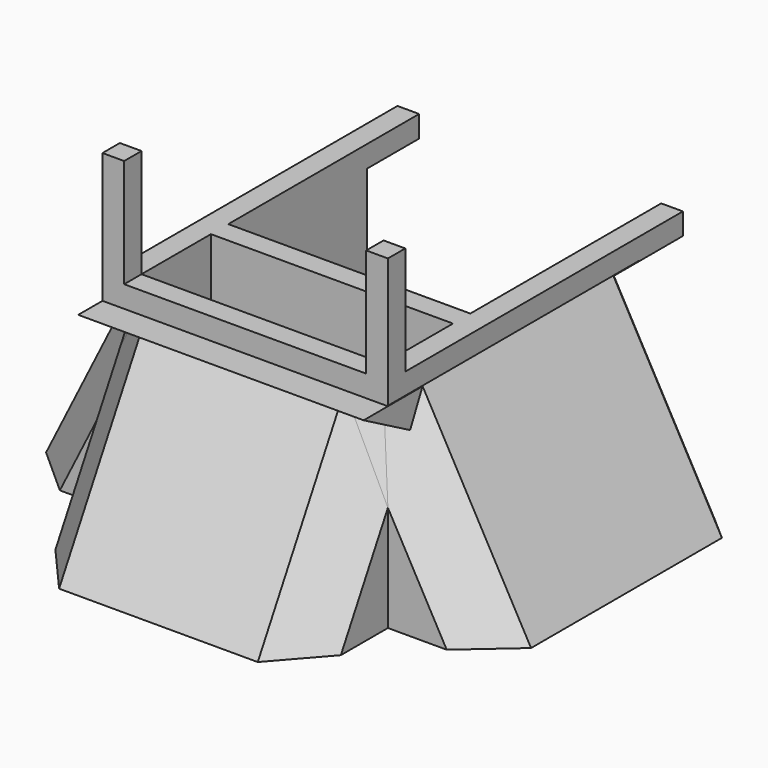
from build123d import *

# Parameters (mm, degrees)
F0_W          = 28.3464
F0_H          = 2.54
F0_W_2        = 2.54
F1_DEPTH      = 43.18
F2_W          = 28.3464
F2_H          = 10.16
F3_DEPTH      = 2.54
F2_W_2        = 2.54
F2_H_2        = 2.54
F4_DEPTH      = 12.7
F5_DEPTH      = 25.4
F6_W          = 33.4264
F6_H          = 22.86
F7_DEPTH      = 12.7
F9_W          = 35.56
F9_H          = 27.94
F10_DEPTH     = 25.4
F11_W         = 35.56
F11_H         = 22.86
F12_DEPTH     = 12.7
F14_W         = 36.8241928518
F14_H         = 28.1280204654
F15_DEPTH     = 25.4
F17_DEPTH     = 12.7
F19_W         = 36.3356121816
F19_H         = 38.6965835933
F20_DEPTH     = 25.4
F21_T4_DEPTH  = 37.4897748093
F21_T10_DEPTH = 37.4897748093
F22_T4_DEPTH  = 41.4622128931
F22_T9_DEPTH  = 41.4622128931
F22_T15_DEPTH = 39.215050137
F22_T21_DEPTH = 39.215050137
F22_T26_DEPTH = 13.1188216118
F23_T4_DEPTH  = 41.4622128931
F23_T9_DEPTH  = 41.4622128931
F23_T14_DEPTH = 39.215050137
F24_W         = 28.3464
F24_H         = 2.54
F25_DEPTH     = 25.4


# Not quite as in the source:
# - a fillet or chamfer that OpenCascade refuses, or shapes differently, is made with other operations: its cross-section is extruded or revolved along the edge and cut away or added


with BuildPart() as f1:
    # F0 (on Front) → F1 (new body)
    with BuildSketch(Plane.XZ):
        with Locations((16.7132, 1.27)):
            Rectangle(F0_W, F0_H)
        with Locations((1.27, 1.27)):
            Rectangle(F0_W_2, F0_H)
        with Locations((32.1564, 1.27)):
            Rectangle(F0_W_2, F0_H)
    extrude(amount=F1_DEPTH)

    # F2 (on face) → F3 (cut)
    with BuildSketch(Plane.XY.offset(2.54)):
        Polygon((30.8864, 0), (2.54, 0), (2.54, -7.62), (2.54, -27.94), (30.8864, -27.94), (30.8864, -7.62), align=None)
        with Locations((16.7132, -35.56)):
            Rectangle(F2_W, F2_H)
    extrude(amount=-F3_DEPTH, mode=Mode.SUBTRACT)

    # F2 (on face) → F4 (join)
    with BuildSketch(Plane.XY.offset(2.54)):
        with Locations((1.27, -41.91)):
            Rectangle(F2_W_2, F2_H_2)
        with Locations((32.1564, -41.91)):
            Rectangle(F2_W_2, F2_H_2)
    extrude(amount=F4_DEPTH)

    # F2 (on face) → F5 (join)
    with BuildSketch(Plane.XY.offset(2.54)):
        Polygon((2.54, -7.62), (0, -7.62), (0, -40.64), (2.54, -40.64), (2.54, -30.48), (2.54, -27.94), align=None)
        Polygon((33.4264, -7.62), (30.8864, -7.62), (30.8864, -27.94), (30.8864, -30.48), (30.8864, -40.64), (33.4264, -40.64), align=None)
        with Locations((16.7132, -41.91)):
            Rectangle(F2_W, F2_H_2)
        with Locations((1.27, -41.91)):
            Rectangle(F2_W_2, F2_H_2)
        with Locations((32.1564, -41.91)):
            Rectangle(F2_W_2, F2_H_2)
    extrude(amount=-F5_DEPTH)

    # F6 (on face) → F7 (join)
    with BuildSketch(Plane.XZ.offset(43.18)):
        with Locations((16.7132, -11.43)):
            Rectangle(F6_W, F6_H)
    extrude(amount=F7_DEPTH)

    # F9 (on 3pt) → F10 (cut)
    with BuildSketch(Plane(origin=(0, -32.9960377358, 18.3311320755), x_dir=(-1, 0, 0), z_dir=(0, 0.8741572761, -0.4856429312))):
        with Locations((-17.78, -36.665337096)):
            Rectangle(F9_W, F9_H)
    extrude(amount=-F10_DEPTH, mode=Mode.SUBTRACT)

    # F11 (on face) → F12 (join)
    with BuildSketch(Plane.YZ.offset(33.4264)):
        with Locations((-25.4, -11.43)):
            Rectangle(F11_W, F11_H)
    extrude(amount=F12_DEPTH)

    # F14 (on 3pt) → F15 (cut)
    with BuildSketch(Plane(origin=(25.5428150943, 0, 14.1904528302), x_dir=(0, -1, 0), z_dir=(-0.8741572761, 0, -0.4856429312))):
        with Locations((24.8448457569, -30.2426330745)):
            Rectangle(F14_W, F14_H)
    extrude(amount=-F15_DEPTH, mode=Mode.SUBTRACT)

    # F16 (on face) → F17 (join)
    with BuildSketch(Plane(origin=(0, 0, 0), x_dir=(0, -1, 0), z_dir=(-1, 0, 0))):
        Polygon((40.64, -22.86), (40.64, 2.54), (7.62, 2.54), (7.62, 0), (7.62, -22.86), align=None)
    extrude(amount=F17_DEPTH)

    # F19 (on 3pt) → F20 (cut)
    with BuildSketch(Plane(origin=(-1.016, 0, 0.508), x_dir=(0, -1, 0), z_dir=(-0.894427191, 0, 0.4472135955))):
        with Locations((25.5430552643, -17.0687864302)):
            Rectangle(F19_W, F19_H)
    extrude(amount=F20_DEPTH, mode=Mode.SUBTRACT)

    # F21: chamfer of 5.08 on 2 edges, made by hand


with BuildPart() as f21_tool2:
    # F21_s3 → F21_t4 (new body)
    with BuildSketch(Plane(origin=(0, -29.228474159, -52.6112534862), x_dir=(1, 0, 0), z_dir=(0, 0.4856429312, 0.8741572761))):
        with BuildLine():
            Line((-0.1436840979, -32.522427085), (5.2236840979, -37.8897952809))
            Line((5.2236840979, -37.8897952809), (5.2236840979, -37.9913952809))
            ThreePointArc((5.2236840979, -37.9913952809), (2.611842049, -37.8477111829), (0, -37.8477111829))
            Line((0, -37.8477111829), (-0.1016, -37.7461111829))
            ThreePointArc((-0.1016, -37.7461111829), (-0.1016, -35.134269134), (-0.2452840979, -32.522427085))
            Line((-0.2452840979, -32.522427085), (-0.1436840979, -32.522427085))
        make_face()
    extrude(amount=F21_T4_DEPTH)

    split(bisect_by=Plane.XY.offset(-22.86), keep=Keep.TOP)

    split(bisect_by=Plane.XZ.offset(40.64), keep=Keep.TOP)


with BuildPart() as f1_1:
    add(f1.part)

    # F21_t1: cut F21_tool2
    add(f21_tool2.part, mode=Mode.SUBTRACT)


with BuildPart() as f21_tool8:
    # F21_s9 → F21_t10 (new body)
    with BuildSketch(Plane(origin=(0, -11.0218300314, -19.8392940565), x_dir=(1, 0, 0), z_dir=(0, -0.4856429312, -0.8741572761))):
        with BuildLine():
            Line((33.5700840979, 32.522427085), (28.2027159021, 37.8897952809))
            Line((28.2027159021, 37.8897952809), (28.2027159021, 37.9913952809))
            ThreePointArc((28.2027159021, 37.9913952809), (30.814557951, 37.8477111829), (33.4264, 37.8477111829))
            Line((33.4264, 37.8477111829), (33.528, 37.7461111829))
            ThreePointArc((33.528, 37.7461111829), (33.528, 35.134269134), (33.6716840979, 32.522427085))
            Line((33.6716840979, 32.522427085), (33.5700840979, 32.522427085))
        make_face()
    extrude(amount=F21_T10_DEPTH)

    split(bisect_by=Plane.XZ.offset(43.18), keep=Keep.TOP)

    split(bisect_by=Plane.XY.offset(-22.86), keep=Keep.TOP)


with BuildPart() as f1_2:
    add(f1_1.part)

    # F21_t7: cut F21_tool8
    add(f21_tool8.part, mode=Mode.SUBTRACT)

    # F22: chamfer of 5.08 on 2 edges, made by hand


with BuildPart() as f22_tool2:
    # F22_s3 → F22_t4 (new body)
    with BuildSketch(Plane(origin=(-17.5264653053, 0, -35.0529306106), x_dir=(0, 1, 0), z_dir=(0.4472135955, 0, 0.894427191))):
        Polygon((-40.64, -3.9440774674), (-35.56, 1.1359225326), (-40.64, 1.1359225326), align=None)
    extrude(amount=F22_T4_DEPTH)

    split(bisect_by=Plane.YZ, keep=Keep.BOTTOM)


with BuildPart() as f1_3:
    add(f1_2.part)

    # F22_t1: cut F22_tool2
    add(f22_tool2.part, mode=Mode.SUBTRACT)


with BuildPart() as f22_tool7:
    # F22_s8 → F22_t9 (new body)
    with BuildSketch(Plane(origin=(-17.5264653053, 0, -35.0529306106), x_dir=(0, 1, 0), z_dir=(0.4472135955, 0, 0.894427191))):
        Polygon((-40.64, -3.9440774674), (-35.56, 1.1359225326), (-40.64, 1.1359225326), align=None)
    extrude(amount=F22_T9_DEPTH)

    split(bisect_by=Plane(origin=(-16.3330555915, -14.2776593863, 7.9320329924), x_dir=(0.6581451817, -0.7528910411, 0), z_dir=(-0.7071067812, -0.6181225378, 0.3434014099)), keep=Keep.TOP)

    split(bisect_by=Plane(origin=(0, -11.0218300314, -19.8392940565), x_dir=(1, 0, 0), z_dir=(0, -0.4856429312, -0.8741572761)), keep=Keep.TOP)


with BuildPart() as f1_4:
    add(f1_3.part)

    # F22_t6: cut F22_tool7
    add(f22_tool7.part, mode=Mode.SUBTRACT)


with BuildPart() as f22_tool13:
    # F22_s14 → F22_t15 (new body)
    with BuildSketch(Plane(origin=(26.9280968005, 0, -48.4705742409), x_dir=(0, 1, 0), z_dir=(-0.4856429312, 0, 0.8741572761))):
        Polygon((-38.1, -29.2199307745), (-43.18, -24.1399307745), (-43.18, -29.2199307745), align=None)
    extrude(amount=F22_T15_DEPTH)

    split(bisect_by=Plane(origin=(33.0462555918, -28.8876247736, 16.0486804298), x_dir=(0.6581451817, 0.7528910411, 0), z_dir=(0.7071067812, -0.6181225378, 0.3434014099)), keep=Keep.TOP)

    split(bisect_by=Plane(origin=(0, -11.0218300314, -19.8392940565), x_dir=(1, 0, 0), z_dir=(0, -0.4856429312, -0.8741572761)), keep=Keep.TOP)


with BuildPart() as f1_5:
    add(f1_4.part)

    # F22_t12: cut F22_tool13
    add(f22_tool13.part, mode=Mode.SUBTRACT)


with BuildPart() as f22_tool19:
    # F22_s20 → F22_t21 (new body)
    with BuildSketch(Plane(origin=(26.9280968005, 0, -48.4705742409), x_dir=(0, 1, 0), z_dir=(-0.4856429312, 0, 0.8741572761))):
        Polygon((-38.1, -29.2199307745), (-43.18, -24.1399307745), (-43.18, -29.2199307745), align=None)
    extrude(amount=F22_T21_DEPTH)

    split(bisect_by=Plane.YZ.offset(33.4264), keep=Keep.TOP)


with BuildPart() as f1_6:
    add(f1_5.part)

    # F22_t18: cut F22_tool19
    add(f22_tool19.part, mode=Mode.SUBTRACT)


with BuildPart() as f22_tool24:
    # F22_s25 → F22_t26 (new body)
    with BuildSketch(Plane(origin=(1.5125219245, 0, -2.7225394641), x_dir=(0, 1, 0), z_dir=(0.4856429312, 0, -0.8741572761))):
        Polygon((-38.1, 29.2199307745), (-43.18, 24.1399307745), (-43.18, 29.2199307745), align=None)
    extrude(amount=F22_T26_DEPTH)

    split(bisect_by=Plane(origin=(33.0462555918, -28.8876247736, 16.0486804298), x_dir=(0.6581451817, 0.7528910411, 0), z_dir=(0.7071067812, -0.6181225378, 0.3434014099)), keep=Keep.TOP)

    split(bisect_by=Plane(origin=(0, -11.0218300314, -19.8392940565), x_dir=(1, 0, 0), z_dir=(0, -0.4856429312, -0.8741572761)), keep=Keep.TOP)


with BuildPart() as f1_7:
    add(f1_6.part)

    # F22_t23: cut F22_tool24
    add(f22_tool24.part, mode=Mode.SUBTRACT)

    # F23: chamfer of 2.54 on 2 edges, made by hand


with BuildPart() as f23_tool2:
    # F23_s3 → F23_t4 (new body)
    with BuildSketch(Plane(origin=(3.9372326527, 0, 7.8744653053), x_dir=(0, 1, 0), z_dir=(-0.4472135955, 0, -0.894427191))):
        Polygon((-10.16, -1.1359225326), (-7.62, 1.4040774674), (-7.62, -1.1359225326), align=None)
    extrude(amount=F23_T4_DEPTH)

    split(bisect_by=Plane.XY, keep=Keep.BOTTOM)


with BuildPart() as f1_8:
    add(f1_7.part)

    # F23_t1: cut F23_tool2
    add(f23_tool2.part, mode=Mode.SUBTRACT)


with BuildPart() as f23_tool7:
    # F23_s8 → F23_t9 (new body)
    with BuildSketch(Plane(origin=(3.9372326527, 0, 7.8744653053), x_dir=(0, 1, 0), z_dir=(-0.4472135955, 0, -0.894427191))):
        Polygon((-10.16, -1.1359225326), (-7.62, 1.4040774674), (-7.62, -1.1359225326), align=None)
    extrude(amount=F23_T9_DEPTH)

    split(bisect_by=Plane.YZ, keep=Keep.BOTTOM)


with BuildPart() as f1_9:
    add(f1_8.part)

    # F23_t6: cut F23_tool7
    add(f23_tool7.part, mode=Mode.SUBTRACT)


with BuildPart() as f23_tool12:
    # F23_s13 → F23_t14 (new body)
    with BuildSketch(Plane(origin=(23.7558408531, 0, -42.7605135355), x_dir=(0, 1, 0), z_dir=(-0.4856429312, 0, 0.8741572761))):
        Polygon((-7.62, -26.6799307745), (-10.16, -29.2199307745), (-7.62, -29.2199307745), align=None)
    extrude(amount=F23_T14_DEPTH)

    split(bisect_by=Plane.XY, keep=Keep.BOTTOM)


with BuildPart() as f1_10:
    add(f1_9.part)

    # F23_t11: cut F23_tool12
    add(f23_tool12.part, mode=Mode.SUBTRACT)

    # F24 (on face) → F25 (join)
    with BuildSketch(Plane.XY.offset(2.54)):
        with Locations((16.7132, -29.21)):
            Rectangle(F24_W, F24_H)
    extrude(amount=-F25_DEPTH)


solid = f1_10.part
